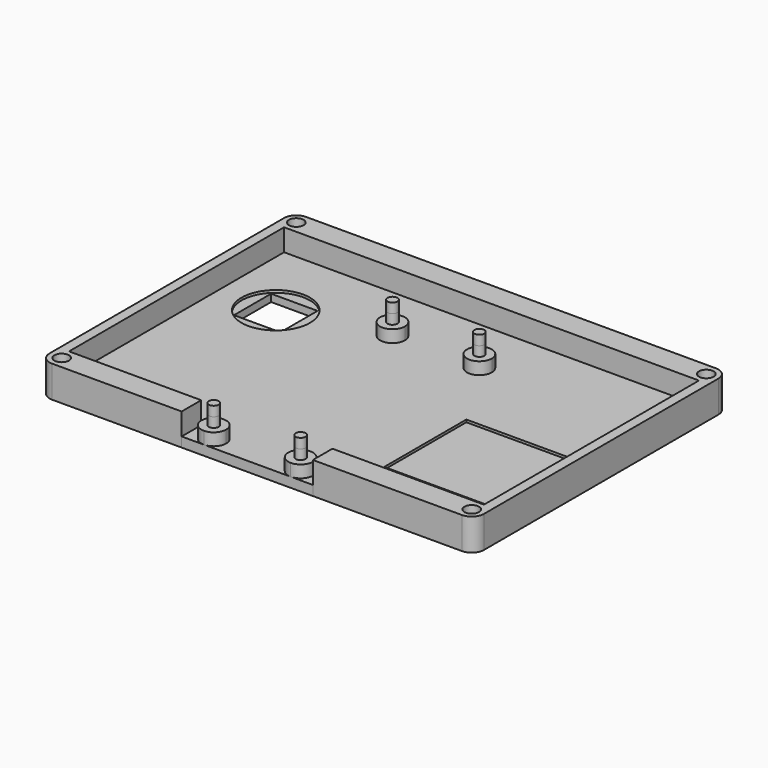
from build123d import *

# Parameters (mm, degrees)
F0_R      = 1.016
F1_DEPTH  = 6.5
F0_R_2    = 1.5
F0_R_3    = 7
F1_FACE_R = 1.016
F2_DEPTH  = 2
F0_W      = 9.5
F0_H      = 9.5
F0_W_2    = 26
F0_H_2    = 21
F3_DEPTH  = 1.5
F4_DEPTH  = 4.5


with BuildPart() as f1:
    # F0 (on Top) → F1 (new body)
    with BuildSketch(Plane.XY):
        with Locations((-10.87, -29.96)):
            Circle(F0_R)
    extrude(amount=F1_DEPTH)


with BuildPart() as f1b:
    # F0 (on Top) → F1, piece 2 (new body)
    with BuildSketch(Plane.XY):
        with Locations((6.91, -29.96)):
            Circle(F0_R)
    extrude(amount=F1_DEPTH)


with BuildPart() as f1c:
    # F0 (on Top) → F1, piece 3 (new body)
    with BuildSketch(Plane.XY):
        with Locations((-10.87, 15.76)):
            Circle(F0_R)
    extrude(amount=F1_DEPTH)


with BuildPart() as f1d:
    # F0 (on Top) → F1, piece 4 (new body)
    with BuildSketch(Plane.XY):
        with Locations((6.91, 15.76)):
            Circle(F0_R)
    extrude(amount=F1_DEPTH)


with BuildPart() as f1e:
    # F0 (on Top) → F1, piece 5 (new body)
    with BuildSketch(Plane.XY):
        with BuildLine():
            Line((-42.45, 27.5), (42.45, 27.5))
            Line((42.45, 27.5), (42.45, 0.5))
            Line((42.45, 0.5), (42.45, -20.5))
            Line((42.45, -20.5), (42.45, -27.5))
            Line((42.45, -27.5), (11.45, -27.5))
            Line((11.45, -27.5), (11.45, -32.5))
            Line((11.45, -32.5), (41.95, -32.5))
            ThreePointArc((41.95, -32.5), (43.717766953, -31.767766953), (44.45, -30))
            Line((44.45, -30), (44.45, -27.5))
            Line((44.45, -27.5), (44.45, 27.5))
            Line((44.45, 27.5), (44.45, 30))
            ThreePointArc((44.45, 30), (43.717766953, 31.767766953), (41.95, 32.5))
            Line((41.95, 32.5), (-41.95, 32.5))
            ThreePointArc((-41.95, 32.5), (-43.717766953, 31.767766953), (-44.45, 30))
            Line((-44.45, 30), (-44.45, 27.5))
            Line((-44.45, 27.5), (-44.45, -27.5))
            Line((-44.45, -27.5), (-44.45, -30))
            ThreePointArc((-44.45, -30), (-43.717766953, -31.767766953), (-41.95, -32.5))
            Line((-41.95, -32.5), (-15.41, -32.5))
            Line((-15.41, -32.5), (-15.41, -27.5))
            Line((-15.41, -27.5), (-42.45, -27.5))
            Line((-42.45, -27.5), (-42.45, 27.5))
        make_face()
        with Locations((-41.95, -30)):
            Circle(F0_R_2, mode=Mode.SUBTRACT)
        with Locations((41.95, -30)):
            Circle(F0_R_2, mode=Mode.SUBTRACT)
        with Locations((-41.95, 30)):
            Circle(F0_R_2, mode=Mode.SUBTRACT)
        with Locations((41.95, 30)):
            Circle(F0_R_2, mode=Mode.SUBTRACT)
    extrude(amount=F1_DEPTH)


with BuildPart() as f2:
    # F0 (on Top) + F1_face (on face) → F2 (new body)
    with BuildSketch(Plane.XY):
        Polygon((42.45, 0.5), (42.45, 27.5), (-42.45, 27.5), (-42.45, -27.5), (-15.41, -27.5), (-15.41, -32.5), (-13.41, -32.5), (-13.41, -29.96), (-13.41, 15.76), (-13.41, 18.3), (-10.87, 18.3), (6.9099999988, 18.3), (9.45, 18.3), (9.45, 15.76), (9.45, -29.96), (9.45, -32.5), (11.45, -32.5), (11.45, -27.5), (42.45, -27.5), (42.45, -20.5), (16.45, -20.5), (16.45, 0.5), align=None)
        with Locations((-30.95, 11)):
            Circle(F0_R_3, mode=Mode.SUBTRACT)
        with BuildLine():
            Line((-13.41, -29.96), (-13.41, -32.5))
            Line((-13.41, -32.5), (-10.87, -32.5))
            ThreePointArc((-10.87, -32.5), (-12.6660512242, -31.7560512242), (-13.41, -29.96))
        make_face()
        with BuildLine():
            ThreePointArc((-8.33, -29.96), (-9.0739487758, -31.7560512242), (-10.87, -32.5))
            Line((-10.87, -32.5), (6.9099999741, -32.5))
            ThreePointArc((6.9099999741, -32.5), (5.1139487849, -28.1639487666), (9.45, -29.96))
            Line((9.45, -29.96), (9.45, 15.76))
            ThreePointArc((9.45, 15.76), (5.1139487762, 13.9639487754), (6.9099999988, 18.3))
            Line((6.9099999988, 18.3), (-10.87, 18.3))
            ThreePointArc((-10.87, 18.3), (-9.0739487758, 17.5560512242), (-8.33, 15.76))
            ThreePointArc((-8.33, 15.76), (-10.87, 13.22), (-13.41, 15.76))
            Line((-13.41, 15.76), (-13.41, -29.96))
            ThreePointArc((-13.41, -29.96), (-10.87, -27.42), (-8.33, -29.96))
        make_face()
        with BuildLine():
            Line((6.9099999741, -32.5), (9.45, -32.5))
            Line((9.45, -32.5), (9.45, -29.96))
            ThreePointArc((9.45, -29.96), (8.7060512151, -31.7560512334), (6.9099999741, -32.5))
        make_face()
        with BuildLine():
            ThreePointArc((6.9099999988, 18.3), (8.7060512238, 17.5560512246), (9.45, 15.76))
            Line((9.45, 15.76), (9.45, 18.3))
            Line((9.45, 18.3), (6.9099999988, 18.3))
        make_face()
        with BuildLine():
            Line((-13.41, 18.3), (-13.41, 15.76))
            ThreePointArc((-13.41, 15.76), (-12.6660512242, 17.5560512242), (-10.87, 18.3))
            Line((-10.87, 18.3), (-13.41, 18.3))
        make_face()
        with BuildLine():
            ThreePointArc((6.9099999988, 18.3), (5.1139487762, 13.9639487754), (9.45, 15.76))
            ThreePointArc((9.45, 15.76), (8.7060512238, 17.5560512246), (6.9099999988, 18.3))
        make_face()
        with Locations((6.91, 15.76)):
            Circle(F0_R, mode=Mode.SUBTRACT)
        with BuildLine():
            ThreePointArc((-13.41, -29.96), (-12.6660512242, -31.7560512242), (-10.87, -32.5))
            ThreePointArc((-10.87, -32.5), (-9.0739487758, -31.7560512242), (-8.33, -29.96))
            ThreePointArc((-8.33, -29.96), (-10.87, -27.42), (-13.41, -29.96))
        make_face()
        with Locations((-10.87, -29.96)):
            Circle(F0_R, mode=Mode.SUBTRACT)
        with BuildLine():
            ThreePointArc((9.45, -29.96), (5.1139487849, -28.1639487666), (6.9099999741, -32.5))
            ThreePointArc((6.9099999741, -32.5), (8.7060512151, -31.7560512334), (9.45, -29.96))
        make_face()
        with Locations((6.91, -29.96)):
            Circle(F0_R, mode=Mode.SUBTRACT)
        with BuildLine():
            ThreePointArc((-10.87, 18.3), (-12.6660512242, 17.5560512242), (-13.41, 15.76))
            ThreePointArc((-13.41, 15.76), (-10.87, 13.22), (-8.33, 15.76))
            ThreePointArc((-8.33, 15.76), (-9.0739487758, 17.5560512242), (-10.87, 18.3))
        make_face()
        with Locations((-10.87, 15.76)):
            Circle(F0_R, mode=Mode.SUBTRACT)
    with BuildSketch(Plane(origin=(-10.87, -29.96, 6.5), x_dir=(1, 0, 0), z_dir=(0, 0, 1))):
        Circle(F1_FACE_R)
        with Locations((17.78, 0)):
            Circle(F1_FACE_R)
        with Locations((0, 45.72)):
            Circle(F1_FACE_R)
        with Locations((17.78, 45.72)):
            Circle(F1_FACE_R)
    extrude(amount=F2_DEPTH)

    # F0 (on Top) → F3 (join)
    with BuildSketch(Plane.XY):
        with Locations((-30.95, 11)):
            Circle(F0_R_3)
        with Locations((-30.95, 11)):
            Rectangle(F0_W, F0_H, mode=Mode.SUBTRACT)
        with Locations((29.45, -10)):
            Rectangle(F0_W_2, F0_H_2)
    extrude(amount=F3_DEPTH)


with BuildPart() as f4:
    # F0 (on Top) → F4 (new body)
    with BuildSketch(Plane.XY):
        with BuildLine():
            ThreePointArc((-10.87, 18.3), (-12.6660512242, 17.5560512242), (-13.41, 15.76))
            ThreePointArc((-13.41, 15.76), (-10.87, 13.22), (-8.33, 15.76))
            ThreePointArc((-8.33, 15.76), (-9.0739487758, 17.5560512242), (-10.87, 18.3))
        make_face()
        with Locations((-10.87, 15.76)):
            Circle(F0_R, mode=Mode.SUBTRACT)
    extrude(amount=F4_DEPTH)


with BuildPart() as f4b:
    # F0 (on Top) → F4, piece 2 (new body)
    with BuildSketch(Plane.XY):
        with BuildLine():
            ThreePointArc((6.9099999988, 18.3), (5.1139487762, 13.9639487754), (9.45, 15.76))
            ThreePointArc((9.45, 15.76), (8.7060512238, 17.5560512246), (6.9099999988, 18.3))
        make_face()
        with Locations((6.91, 15.76)):
            Circle(F0_R, mode=Mode.SUBTRACT)
    extrude(amount=F4_DEPTH)


with BuildPart() as f4c:
    # F0 (on Top) → F4, piece 3 (new body)
    with BuildSketch(Plane.XY):
        with BuildLine():
            ThreePointArc((9.45, -29.96), (5.1139487849, -28.1639487666), (6.9099999741, -32.5))
            ThreePointArc((6.9099999741, -32.5), (8.7060512151, -31.7560512334), (9.45, -29.96))
        make_face()
        with Locations((6.91, -29.96)):
            Circle(F0_R, mode=Mode.SUBTRACT)
    extrude(amount=F4_DEPTH)


with BuildPart() as f4d:
    # F0 (on Top) → F4, piece 4 (new body)
    with BuildSketch(Plane.XY):
        with BuildLine():
            ThreePointArc((-13.41, -29.96), (-12.6660512242, -31.7560512242), (-10.87, -32.5))
            ThreePointArc((-10.87, -32.5), (-9.0739487758, -31.7560512242), (-8.33, -29.96))
            ThreePointArc((-8.33, -29.96), (-10.87, -27.42), (-13.41, -29.96))
        make_face()
        with Locations((-10.87, -29.96)):
            Circle(F0_R, mode=Mode.SUBTRACT)
    extrude(amount=F4_DEPTH)


solid = Compound([f1.part, f1b.part, f1c.part, f1d.part, f1e.part, f2.part, f4.part, f4b.part, f4c.part, f4d.part])
